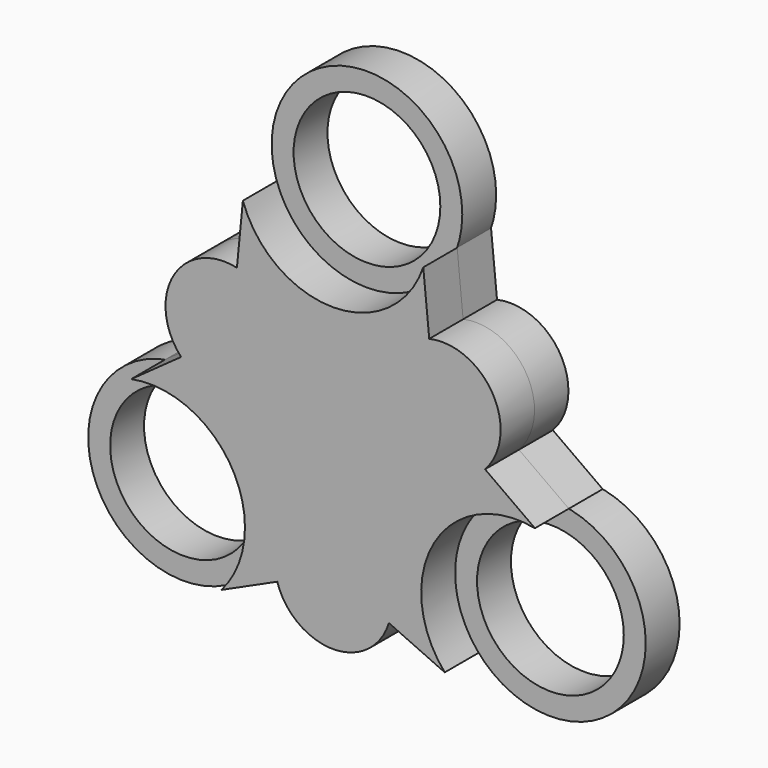
from build123d import *

# Parameters (mm, degrees)
F0_R     = 14.2875
F0_R_2   = 10.9982
F2_DEPTH = 6.35
F1_W     = 0.4390429688
F1_H     = 3.7777539063
F1_R     = 14.2875
F1_W_2   = 0.3297629937
F1_H_2   = 2.8374522002
F5_DEPTH = 6.35
F7_DEPTH = 6.35
F8_DEPTH = 6.35


with BuildPart() as f2:
    # F0 (on Front) → F2 (new body)
    with BuildSketch(Plane.XZ):
        with Locations((0, 31.75)):
            Circle(F0_R)
        with Locations((0, 31.75)):
            Circle(F0_R_2, mode=Mode.SUBTRACT)
    extrude(amount=F2_DEPTH)


with BuildPart() as f2b:
    # F0 (on Front) → F2, piece 2 (new body)
    with BuildSketch(Plane.XZ):
        Circle(F0_R)
        Circle(F0_R_2, mode=Mode.SUBTRACT)
    extrude(amount=F2_DEPTH)


with BuildPart() as f2c:
    # F0 (on Front) → F2, piece 3 (new body)
    with BuildSketch(Plane.XZ):
        with Locations((-27.4963065702, -15.875)):
            Circle(F0_R)
        with Locations((-27.4963065702, -15.875)):
            Circle(F0_R_2, mode=Mode.SUBTRACT)
    extrude(amount=F2_DEPTH)


with BuildPart() as f2d:
    # F0 (on Front) → F2, piece 4 (new body)
    with BuildSketch(Plane.XZ):
        with Locations((27.4963065702, -15.875)):
            Circle(F0_R)
        with Locations((27.4963065702, -15.875)):
            Circle(F0_R_2, mode=Mode.SUBTRACT)
    extrude(amount=F2_DEPTH)


with BuildPart() as f2e:
    # F1 (on Front) → F2, piece 5 (new body)
    with BuildSketch(Plane.XZ):
        with BuildLine():
            ThreePointArc((13.5206938879, 27.1322632123), (0, 17.4625), (-13.5206938879, 27.1322632123))
            ThreePointArc((-13.5206938879, 27.1322632123), (-15.305469781, 8.8366170981), (-30.257576148, -1.8568672225))
            ThreePointArc((-30.257576148, -1.8568672225), (-18.4221394691, -4.8390520266), (-13.2088065702, -15.875))
            ThreePointArc((-13.2088065702, -15.875), (-14.1198733557, -20.8953277493), (-16.7368822601, -25.2753959899))
            ThreePointArc((-16.7368822601, -25.2753959899), (-11.342771298, -20.7856162625), (-4.8176097302, -18.2016616216))
            Line((-4.8176097302, -18.2016616216), (-5.5088278546, -18.2016616216))
            Line((-5.5088278546, -18.2016616216), (-5.5088278546, -14.4239077154))
            Line((-5.5088278546, -14.4239077154), (-3.4029098859, -14.4239077154))
            Line((-3.4029098859, -14.4239077154), (-3.4029098859, -14.814168132))
            Line((-3.4029098859, -14.814168132), (-5.0697848859, -14.814168132))
            Line((-5.0697848859, -14.814168132), (-5.0697848859, -16.0312514654))
            Line((-5.0697848859, -16.0312514654), (-3.5037822817, -16.0312514654))
            Line((-3.5037822817, -16.0312514654), (-3.5037822817, -16.4190314133))
            Line((-3.5037822817, -16.4190314133), (-5.0697848859, -16.4190314133))
            Line((-5.0697848859, -16.4190314133), (-5.0697848859, -17.8089207362))
            Line((-5.0697848859, -17.8089207362), (-3.4029098859, -17.8089207362))
            Line((-3.4029098859, -17.8089207362), (-3.4029098859, -17.9352920139))
            ThreePointArc((-3.4029098859, -17.9352920139), (-2.9850761481, -17.8746117561), (-2.5661650942, -17.821879839))
            Line((-2.5661650942, -17.821879839), (-2.5661650942, -14.4239077154))
            Line((-2.5661650942, -14.4239077154), (-2.0700713442, -14.4239077154))
            Line((-2.0700713442, -14.4239077154), (-0.0104554588, -17.5815444341))
            Line((-0.0104554588, -17.5815444341), (0.0102151141, -17.5815444341))
            add(Edge.make_bspline(
                [(0.0102151141, -17.5815444341), (0.0052541766, -17.5120913091), (-0.0129359276, -17.1334064133)],
                knots=[0, 0, 0, 1, 1, 1], degree=2))
            add(Edge.make_bspline(
                [(-0.0129359276, -17.1334064133), (-0.0311260317, -16.7547215175), (-0.0261650942, -16.5918374029)],
                knots=[0, 0, 0, 1, 1, 1], degree=2))
            Line((-0.0261650942, -16.5918374029), (-0.0261650942, -14.4239077154))
            Line((-0.0261650942, -14.4239077154), (0.3847658954, -14.4239077154))
            Line((0.3847658954, -14.4239077154), (0.3847658954, -17.6765650374))
            ThreePointArc((0.3847658954, -17.6765650374), (0.9042579175, -17.6916373697), (1.4232554787, -17.7188525809))
            Line((1.4232554787, -17.7188525809), (1.4232554787, -14.4239077154))
            Line((1.4232554787, -14.4239077154), (1.9193492287, -14.4239077154))
            Line((1.9193492287, -14.4239077154), (3.9789651141, -17.5815444341))
            Line((3.9789651141, -17.5815444341), (3.999635687, -17.5815444341))
            add(Edge.make_bspline(
                [(3.999635687, -17.5815444341), (3.9946747495, -17.5120913091), (3.9764846454, -17.1334064133)],
                knots=[0, 0, 0, 1, 1, 1], degree=2))
            add(Edge.make_bspline(
                [(3.9764846454, -17.1334064133), (3.9582945412, -16.7547215175), (3.9632554787, -16.5918374029)],
                knots=[0, 0, 0, 1, 1, 1], degree=2))
            Line((3.9632554787, -16.5918374029), (3.9632554787, -14.4239077154))
            Line((3.9632554787, -14.4239077154), (4.3741864683, -14.4239077154))
            Line((4.3741864683, -14.4239077154), (4.3741864683, -18.1079354893))
            ThreePointArc((4.3741864683, -18.1079354893), (11.1473058727, -20.6709567816), (16.7368822601, -25.2753959899))
            ThreePointArc((16.7368822601, -25.2753959899), (15.1229686136, -8.73125), (30.257576148, -1.8568672225))
            ThreePointArc((30.257576148, -1.8568672225), (15.305469781, 8.8366170981), (13.5206938879, 27.1322632123))
        make_face()
        Polygon((-7.2740947817, -14.814168132), (-7.2740947817, -18.2016616216), (-7.7131377505, -18.2016616216), (-7.7131377505, -14.814168132), (-8.9095505109, -14.814168132), (-8.9095505109, -14.4239077154), (-6.0776820213, -14.4239077154), (-6.0776820213, -14.814168132), align=None, mode=Mode.SUBTRACT)
        with Locations((5.632197536, -16.3127846685)):
            Rectangle(F1_W, F1_H, mode=Mode.SUBTRACT)
        with BuildLine():
            add(Edge.make_bspline(
                [(8.7960354266, -16.5662058925), (9.0192776141, -16.80929183), (9.0192776141, -17.196244955)],
                knots=[0, 0, 0, 1, 1, 1], degree=2))
            add(Edge.make_bspline(
                [(9.0192776141, -17.196244955), (9.0192776141, -17.6948191737), (8.6575425881, -17.9742853195)],
                knots=[0, 0, 0, 1, 1, 1], degree=2))
            add(Edge.make_bspline(
                [(8.6575425881, -17.9742853195), (8.295807562, -18.2537514654), (7.6756903745, -18.2537514654)],
                knots=[0, 0, 0, 1, 1, 1], degree=2))
            add(Edge.make_bspline(
                [(7.6756903745, -18.2537514654), (7.0043101662, -18.2537514654), (6.6421617287, -18.0801186529)],
                knots=[0, 0, 0, 1, 1, 1], degree=2))
            Line((6.6421617287, -18.0801186529), (6.6421617287, -17.6567853195))
            add(Edge.make_bspline(
                [(6.6421617287, -17.6567853195), (6.8753257912, -17.7543504237), (7.1490041766, -17.811401205)],
                knots=[0, 0, 0, 1, 1, 1], degree=2))
            add(Edge.make_bspline(
                [(7.1490041766, -17.811401205), (7.422682562, -17.8684519862), (7.6914000099, -17.8684519862)],
                knots=[0, 0, 0, 1, 1, 1], degree=2))
            add(Edge.make_bspline(
                [(7.6914000099, -17.8684519862), (8.1304429787, -17.8684519862), (8.3528583433, -17.7018471685)],
                knots=[0, 0, 0, 1, 1, 1], degree=2))
            add(Edge.make_bspline(
                [(8.3528583433, -17.7018471685), (8.5752737079, -17.5352423508), (8.5752737079, -17.2375861008)],
                knots=[0, 0, 0, 1, 1, 1], degree=2))
            add(Edge.make_bspline(
                [(8.5752737079, -17.2375861008), (8.5752737079, -17.0416290695), (8.4963121193, -16.9163653977)],
                knots=[0, 0, 0, 1, 1, 1], degree=2))
            add(Edge.make_bspline(
                [(8.4963121193, -16.9163653977), (8.4173505308, -16.7911017258), (8.2325556089, -16.684854981)],
                knots=[0, 0, 0, 1, 1, 1], degree=2))
            add(Edge.make_bspline(
                [(8.2325556089, -16.684854981), (8.047760687, -16.5786082362), (7.670729437, -16.4446629237)],
                knots=[0, 0, 0, 1, 1, 1], degree=2))
            add(Edge.make_bspline(
                [(7.670729437, -16.4446629237), (7.1440432391, -16.2561472987), (6.9179071714, -15.9977651373)],
                knots=[0, 0, 0, 1, 1, 1], degree=2))
            add(Edge.make_bspline(
                [(6.9179071714, -15.9977651373), (6.6917711037, -15.7393829758), (6.6917711037, -15.3234910487)],
                knots=[0, 0, 0, 1, 1, 1], degree=2))
            add(Edge.make_bspline(
                [(6.6917711037, -15.3234910487), (6.6917711037, -14.8869285487), (7.0196063901, -14.6285463873)],
                knots=[0, 0, 0, 1, 1, 1], degree=2))
            add(Edge.make_bspline(
                [(7.0196063901, -14.6285463873), (7.3474416766, -14.3701642258), (7.8881838641, -14.3701642258)],
                knots=[0, 0, 0, 1, 1, 1], degree=2))
            add(Edge.make_bspline(
                [(7.8881838641, -14.3701642258), (8.4512502704, -14.3701642258), (8.9241929787, -14.576869955)],
                knots=[0, 0, 0, 1, 1, 1], degree=2))
            Line((8.9241929787, -14.576869955), (8.7869403745, -14.9588621425))
            add(Edge.make_bspline(
                [(8.7869403745, -14.9588621425), (8.3189586037, -14.7629051112), (7.8774351662, -14.7629051112)],
                knots=[0, 0, 0, 1, 1, 1], degree=2))
            add(Edge.make_bspline(
                [(7.8774351662, -14.7629051112), (7.5285158954, -14.7629051112), (7.3321454526, -14.9125600591)],
                knots=[0, 0, 0, 1, 1, 1], degree=2))
            add(Edge.make_bspline(
                [(7.3321454526, -14.9125600591), (7.1357750099, -15.062215007), (7.1357750099, -15.3284519862)],
                knots=[0, 0, 0, 1, 1, 1], degree=2))
            add(Edge.make_bspline(
                [(7.1357750099, -15.3284519862), (7.1357750099, -15.5244090175), (7.2081220151, -15.6500861008)],
                knots=[0, 0, 0, 1, 1, 1], degree=2))
            add(Edge.make_bspline(
                [(7.2081220151, -15.6500861008), (7.2804690204, -15.7757631841), (7.452448187, -15.8803562831)],
                knots=[0, 0, 0, 1, 1, 1], degree=2))
            add(Edge.make_bspline(
                [(7.452448187, -15.8803562831), (7.6244273537, -15.984949382), (7.978307562, -16.1114532883)],
                knots=[0, 0, 0, 1, 1, 1], degree=2))
            add(Edge.make_bspline(
                [(7.978307562, -16.1114532883), (8.5727932391, -16.323119955), (8.7960354266, -16.5662058925)],
                knots=[0, 0, 0, 1, 1, 1], degree=2))
        make_face(mode=Mode.SUBTRACT)
        Circle(F1_R, mode=Mode.SUBTRACT)
        Polygon((-3.553615096, 16.0265346236), (-2.3699460451, 14.4218122587), (-2.758085162, 14.4218122587), (-3.7920877694, 15.7979983115), (-4.0895575886, 15.534063712), (-4.0895575886, 14.4218122587), (-4.4193205823, 14.4218122587), (-4.4193205823, 17.2592644588), (-4.0895575886, 17.2592644588), (-4.0895575886, 15.8520272766), (-2.8027987883, 17.2592644588), (-2.4127966036, 17.2592644588), align=None, mode=Mode.SUBTRACT)
        with Locations((-1.8150623636, 15.8405383587)):
            Rectangle(F1_W_2, F1_H_2, mode=Mode.SUBTRACT)
        Polygon((0.0011181922, 16.9661417977), (0.0011181922, 14.4218122587), (-0.3286448015, 14.4218122587), (-0.3286448015, 16.9661417977), (-1.2272644849, 16.9661417977), (-1.2272644849, 17.2592644588), (0.8997378756, 17.2592644588), (0.8997378756, 16.9661417977), align=None, mode=Mode.SUBTRACT)
        with BuildLine():
            add(Edge.make_bspline(
                [(2.7603215464, 15.6501949358), (2.9279976449, 15.4676142952), (2.9279976449, 15.1769757245)],
                knots=[0, 0, 0, 1, 1, 1], degree=2))
            add(Edge.make_bspline(
                [(2.9279976449, 15.1769757245), (2.9279976449, 14.8024991045), (2.6563002631, 14.5925934701)],
                knots=[0, 0, 0, 1, 1, 1], degree=2))
            add(Edge.make_bspline(
                [(2.6563002631, 14.5925934701), (2.3846028812, 14.3826878357), (1.918835941, 14.3826878357)],
                knots=[0, 0, 0, 1, 1, 1], degree=2))
            add(Edge.make_bspline(
                [(1.918835941, 14.3826878357), (1.4145656003, 14.3826878357), (1.1425577072, 14.513102579)],
                knots=[0, 0, 0, 1, 1, 1], degree=2))
            Line((1.1425577072, 14.513102579), (1.1425577072, 14.8310661435))
            add(Edge.make_bspline(
                [(1.1425577072, 14.8310661435), (1.3176860767, 14.7577854782), (1.523244553, 14.7149349197)],
                knots=[0, 0, 0, 1, 1, 1], degree=2))
            add(Edge.make_bspline(
                [(1.523244553, 14.7149349197), (1.7288030293, 14.6720843612), (1.9306353701, 14.6720843612)],
                knots=[0, 0, 0, 1, 1, 1], degree=2))
            add(Edge.make_bspline(
                [(1.9306353701, 14.6720843612), (2.2603983638, 14.6720843612), (2.4274534397, 14.7972204125)],
                knots=[0, 0, 0, 1, 1, 1], degree=2))
            add(Edge.make_bspline(
                [(2.4274534397, 14.7972204125), (2.5945085157, 14.9223564638), (2.5945085157, 15.1459245951)],
                knots=[0, 0, 0, 1, 1, 1], degree=2))
            add(Edge.make_bspline(
                [(2.5945085157, 15.1459245951), (2.5945085157, 15.2931069483), (2.5352008586, 15.3871918702)],
                knots=[0, 0, 0, 1, 1, 1], degree=2))
            add(Edge.make_bspline(
                [(2.5352008586, 15.3871918702), (2.4758932015, 15.4812767921), (2.3370946533, 15.5610781946)],
                knots=[0, 0, 0, 1, 1, 1], degree=2))
            add(Edge.make_bspline(
                [(2.3370946533, 15.5610781946), (2.1982961051, 15.640879597), (1.9151098054, 15.7414852561)],
                knots=[0, 0, 0, 1, 1, 1], degree=2))
            add(Edge.make_bspline(
                [(1.9151098054, 15.7414852561), (1.5195184175, 15.883078406), (1.34966874, 16.0771479644)],
                knots=[0, 0, 0, 1, 1, 1], degree=2))
            add(Edge.make_bspline(
                [(1.34966874, 16.0771479644), (1.1798190624, 16.2712175228), (1.1798190624, 16.5835918841)],
                knots=[0, 0, 0, 1, 1, 1], degree=2))
            add(Edge.make_bspline(
                [(1.1798190624, 16.5835918841), (1.1798190624, 16.9114918101), (1.4260545182, 17.1055613685)],
                knots=[0, 0, 0, 1, 1, 1], degree=2))
            add(Edge.make_bspline(
                [(1.4260545182, 17.1055613685), (1.6722899739, 17.299630927), (2.0784387458, 17.299630927)],
                knots=[0, 0, 0, 1, 1, 1], degree=2))
            add(Edge.make_bspline(
                [(2.0784387458, 17.299630927), (2.5013551276, 17.299630927), (2.8565800474, 17.1443752802)],
                knots=[0, 0, 0, 1, 1, 1], degree=2))
            Line((2.8565800474, 17.1443752802), (2.7534902979, 16.857462845))
            add(Edge.make_bspline(
                [(2.7534902979, 16.857462845), (2.4019915137, 17.0046451981), (2.0703654522, 17.0046451981)],
                knots=[0, 0, 0, 1, 1, 1], degree=2))
            add(Edge.make_bspline(
                [(2.0703654522, 17.0046451981), (1.8082939205, 17.0046451981), (1.6608010561, 16.8922401099)],
                knots=[0, 0, 0, 1, 1, 1], degree=2))
            add(Edge.make_bspline(
                [(1.6608010561, 16.8922401099), (1.5133081916, 16.7798350216), (1.5133081916, 16.5798657486)],
                knots=[0, 0, 0, 1, 1, 1], degree=2))
            add(Edge.make_bspline(
                [(1.5133081916, 16.5798657486), (1.5133081916, 16.4326833955), (1.567647668, 16.3382879622)],
                knots=[0, 0, 0, 1, 1, 1], degree=2))
            add(Edge.make_bspline(
                [(1.567647668, 16.3382879622), (1.6219871444, 16.243892529), (1.7511598425, 16.1653331718)],
                knots=[0, 0, 0, 1, 1, 1], degree=2))
            add(Edge.make_bspline(
                [(1.7511598425, 16.1653331718), (1.8803325406, 16.0867738145), (2.1461302078, 15.9917573587)],
                knots=[0, 0, 0, 1, 1, 1], degree=2))
            add(Edge.make_bspline(
                [(2.1461302078, 15.9917573587), (2.5926454479, 15.8327755764), (2.7603215464, 15.6501949358)],
                knots=[0, 0, 0, 1, 1, 1], degree=2))
        make_face(mode=Mode.SUBTRACT)
        Polygon((5.6337930566, 14.4218122587), (5.2922306337, 14.4218122587), (4.9388687817, 15.3241580776), (3.8017764249, 15.3241580776), (3.4527617309, 14.4218122587), (3.1186515791, 14.4218122587), (4.2402183713, 17.271063888), (4.5178154677, 17.271063888), align=None, mode=Mode.SUBTRACT)
    extrude(amount=F2_DEPTH)

    # F4 (on Front) → F5 (join)
    with BuildSketch(Plane.XZ):
        with BuildLine():
            ThreePointArc((-15.305469781, 8.8366170981), (-12.4328863407, 17.7912682301), (-13.5206938879, 27.1322632123))
            Line((-13.5206938879, 27.1322632123), (-15.305469781, 8.8366170981))
        make_face()
        with BuildLine():
            ThreePointArc((-30.257576148, -1.8568672225), (-21.6241334232, 1.8715612984), (-15.305469781, 8.8366170981))
            Line((-15.305469781, 8.8366170981), (-30.257576148, -1.8568672225))
        make_face()
        with BuildLine():
            Line((15.305469781, 8.8366170981), (13.5206938879, 27.1322632123))
            ThreePointArc((13.5206938879, 27.1322632123), (12.4328863407, 17.7912682301), (15.305469781, 8.8366170981))
        make_face()
        with BuildLine():
            Line((30.257576148, -1.8568672225), (15.305469781, 8.8366170981))
            ThreePointArc((15.305469781, 8.8366170981), (21.6241334232, 1.8715612984), (30.257576148, -1.8568672225))
        make_face()
        with BuildLine():
            ThreePointArc((13.5206938879, 27.1322632123), (0, 17.4625), (-13.5206938879, 27.1322632123))
            ThreePointArc((-13.5206938879, 27.1322632123), (-12.4328863407, 17.7912682301), (-15.305469781, 8.8366170981))
            ThreePointArc((-15.305469781, 8.8366170981), (-21.6241334232, 1.8715612984), (-30.257576148, -1.8568672225))
            ThreePointArc((-30.257576148, -1.8568672225), (-18.4221394691, -4.8390520266), (-13.2088065702, -15.875))
            ThreePointArc((-13.2088065702, -15.875), (-14.1198733557, -20.8953277493), (-16.7368822601, -25.2753959899))
            Line((-16.7368822601, -25.2753959899), (0, -17.6732341963))
            Line((0, -17.6732341963), (16.7368822601, -25.2753959899))
            ThreePointArc((16.7368822601, -25.2753959899), (15.1229686136, -8.73125), (30.257576148, -1.8568672225))
            ThreePointArc((30.257576148, -1.8568672225), (21.6241334232, 1.8715612984), (15.305469781, 8.8366170981))
            ThreePointArc((15.305469781, 8.8366170981), (12.4328863407, 17.7912682301), (13.5206938879, 27.1322632123))
        make_face()
    extrude(amount=F5_DEPTH)

    # F6 (on Front) → F7 (join)
    with BuildSketch(Plane.XZ):
        with BuildLine():
            Line((-15.305469781, 8.8366170981), (-14.4130818345, 17.9844401552))
            ThreePointArc((-14.4130818345, 17.9844401552), (-23.9447381252, 13.8245010023), (-22.7815229645, 3.4898749378))
            Line((-22.7815229645, 3.4898749378), (-15.305469781, 8.8366170981))
        make_face()
        with BuildLine():
            ThreePointArc((22.7815229645, 3.4898749378), (23.9447381252, 13.8245010023), (14.4130818345, 17.9844401552))
            Line((14.4130818345, 17.9844401552), (15.305469781, 8.8366170981))
            Line((15.305469781, 8.8366170981), (22.7815229645, 3.4898749378))
        make_face()
        with BuildLine():
            Line((0, -17.6732341963), (-8.36844113, -21.4743150931))
            ThreePointArc((-8.36844113, -21.4743150931), (0, -27.6490020045), (8.36844113, -21.4743150931))
            Line((8.36844113, -21.4743150931), (0, -17.6732341963))
        make_face()
    extrude(amount=F7_DEPTH)


with BuildPart() as f8:
    # F8 (new): a face of the model
    f8_faces = [f2e.part.faces().sort_by_distance(p)[0] for p in [
        (0, -6.35, 0),
    ]]
    extrude(f8_faces, amount=F8_DEPTH)


solid = Compound([f2.part, f2b.part, f2c.part, f2d.part, f2e.part, f8.part])
